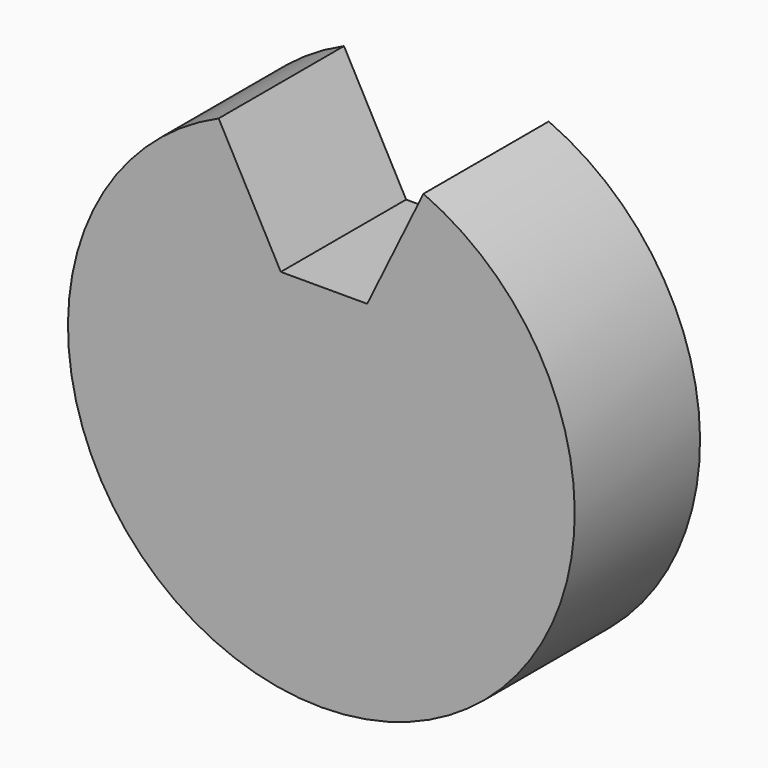
from build123d import *

# Parameters (mm, degrees)
F1_DEPTH = 34.544


# Not quite as in the source:
# - a feature names something its author has since deleted; it is built from what else it names


with BuildPart() as f1:
    # F0 (on Front) → F1 (new body)
    with BuildSketch(Plane.XZ):
        with BuildLine():
            ThreePointArc((-22.5633601832, 19.345696453), (-30.3903128941, -78.5802494572), (55.9621573201, -31.7400641561))
            ThreePointArc((55.9621573201, -31.7400641561), (46.8836011402, -1.2081258561), (22.5978317526, 19.4030566408))
            Line((22.5978317526, 19.4030566408), (10.1926827312, -5.9961574152))
            Line((10.1926827312, -5.9961574152), (-8.8573172688, -5.9961574152))
            Line((-8.8573172688, -5.9961574152), (-22.5633601832, 19.345696453))
        make_face()
    extrude(amount=-F1_DEPTH)


solid = f1.part
